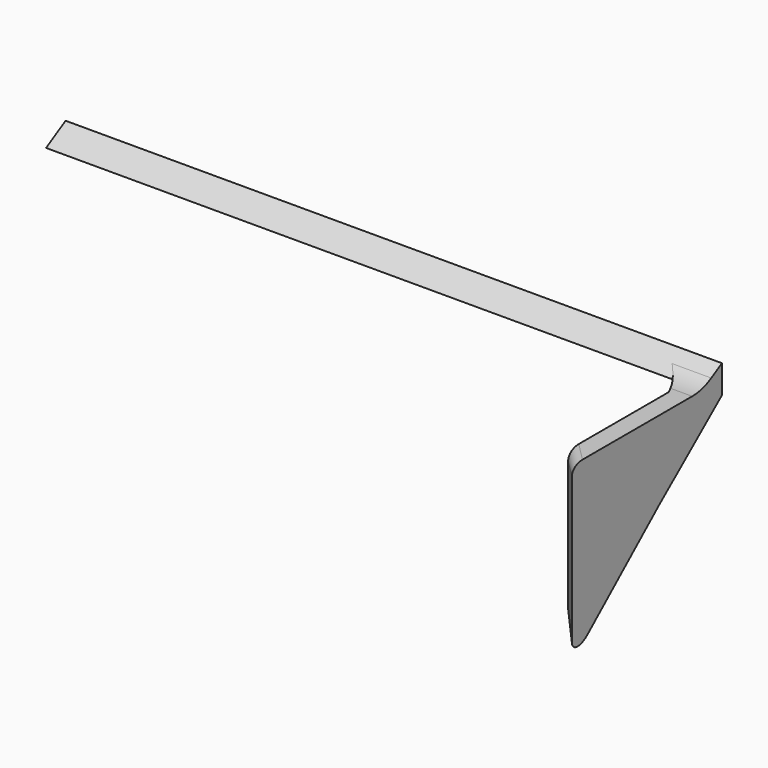
from build123d import *

# Parameters (mm, degrees)
F0_W      = 10
F0_H      = 10
F1_DEPTH  = 2
F3_DEPTH  = 60
F5_DEPTH  = 2
F7_DEPTH  = 2
F9_SIZE   = 1
F10_R     = 5.08
F11_DEPTH = 2.9920059478
F12_DEPTH = 10
F13_DEPTH = 10
F14_DEPTH = 10
F16_DEPTH = 2
F17_SIZE  = 1.99999
F18_R     = 1


# Not quite as in the source:
# - a fillet or chamfer is up to 0.001 mm smaller than in the source, because OpenCascade refuses the exact size


with BuildPart() as f1:
    # F0 (on Right) → F1 (new body)
    with BuildSketch(Plane.YZ):
        with Locations((-5, -5)):
            Rectangle(F0_W, F0_H)
    extrude(amount=F1_DEPTH)

    # F2 (on face) → F3 (join)
    with BuildSketch(Plane.YZ.offset(2)):
        Polygon((0, -3), (0, 0), (-2.5980762114, -1.5), align=None)
    extrude(amount=-F3_DEPTH)

    # F4 (on face) → F5 (cut, through all)
    with BuildSketch(Plane(origin=(0, 0, 0), x_dir=(0, -1, 0), z_dir=(-1, 0, 0))):
        Polygon((10, 0), (0, 0), (2.5980762114, -1.5), align=None)
    extrude(amount=-F5_DEPTH, mode=Mode.SUBTRACT)

    # F6 (on face) → F7 (cut, through all)
    with BuildSketch(Plane.YZ.offset(2)):
        Polygon((-10, -1.5), (-2.5980762114, -1.5), (-10, 0), align=None)
    extrude(amount=-F7_DEPTH, mode=Mode.SUBTRACT)

    # F9
    f9_edges = [f1.edges().sort_by_distance(p)[0] for p in [
        (0, -1.299038, -2.25),
    ]]
    chamfer(f9_edges, length=F9_SIZE)

    # F10
    f10_edges = [f1.edges().sort_by_distance(p)[0] for p in [
        (1, -2.598076, -1.5),
    ]]
    fillet(f10_edges, radius=F10_R)

    # F8 (on face) → F11 (cut, through all)
    with BuildSketch(Plane.YZ.offset(2)):
        Polygon((0, -10), (0, -3.0103854369), (-8.4680961445, -10), align=None)
    extrude(amount=-F11_DEPTH, mode=Mode.SUBTRACT)

    # F12 (add): a face of the model
    f12_faces = [f1.faces().sort_by_distance(p)[0] for p in [
        (-58, -0.8660254038, -1.5),
    ]]
    extrude(f12_faces, amount=F12_DEPTH)

    # F13 (add): a face of the model
    f13_faces = [f1.faces().sort_by_distance(p)[0] for p in [
        (1, -10, -5.75),
    ]]
    extrude(f13_faces, amount=F13_DEPTH)

    # F14 (add): a face of the model
    f14_faces = [f1.faces().sort_by_distance(p)[0] for p in [
        (1, -14.2340480722, -10),
    ]]
    extrude(f14_faces, amount=F14_DEPTH)

    # F15 (on face) → F16 (cut, through all)
    with BuildSketch(Plane.YZ.offset(2)):
        Polygon((-8.4680961445, -20), (-8.4680961445, -10), (-20, -20), align=None)
    extrude(amount=-F16_DEPTH, mode=Mode.SUBTRACT)

    # F17 (size 2 in the source; OpenCascade refuses exactly that, so slightly less here)
    f17_edges = [f1.edges().sort_by_distance(p)[0] for p in [
        (0, -20, -10.75),
    ]]
    chamfer(f17_edges, length=F17_SIZE)

    # F18
    f18_edges = [f1.edges().sort_by_distance(p)[0] for p in [
        (0.999995, -19.000005, -1.5),
        (0.999995, -19.000005, -19.132845),
    ]]
    fillet(f18_edges, radius=F18_R)


solid = f1.part
